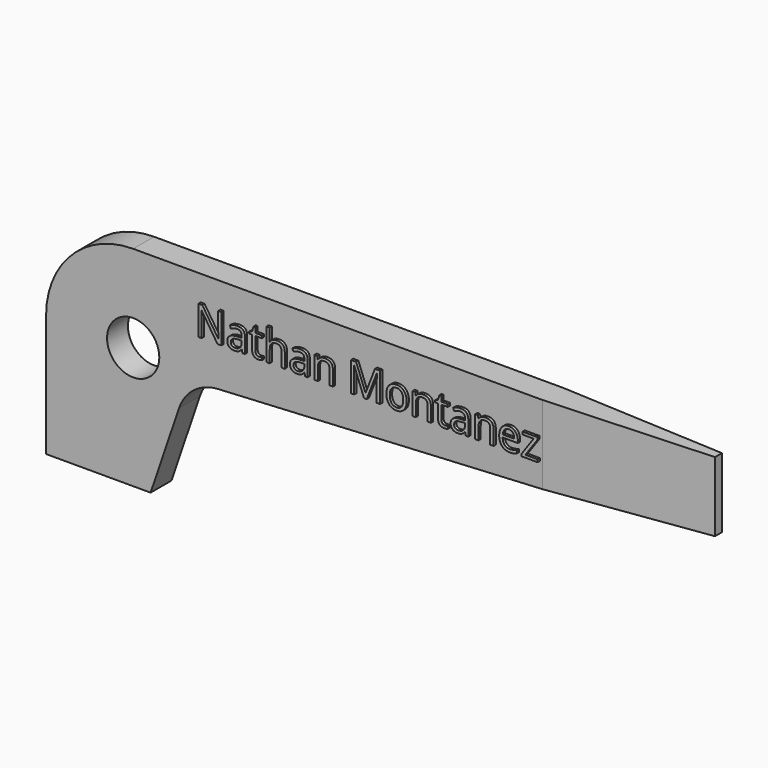
from build123d import *

# Parameters (mm, degrees)
F1_DEPTH     = 2.38125
F2_R         = 2.38125
F3_DEPTH     = 25.4
F5_DEPTH     = 25.4
F6_TEXT_SIZE = 3.7509316959
F7_DEPTH     = 0.254


# Not quite as in the source:
# - Text() gives the source's letters only with a copy of the font that has no kerning and outlines rounded to 1/6400 em; it was checked with that copy


with BuildPart() as f1:
    # F0 (on Front) → F1 (new body)
    with BuildSketch(Plane.XZ):
        with BuildLine():
            Line((60.325, 19.05), (7.9375, 19.05))
            ThreePointArc((7.9375, 19.05), (2.3248399243, 16.7251600757), (0, 11.1125))
            Line((0, 11.1125), (0, 0))
            Line((0, 0), (9.525, 0))
            Line((9.525, 0), (12.1173647876, 7.6271664624))
            ThreePointArc((12.1173647876, 7.6271664624), (13.4786145605, 9.5135918491), (15.6631963617, 10.3130942181))
            Line((15.6631963617, 10.3130942181), (60.325, 12.7))
            Line((60.325, 12.7), (60.325, 19.05))
        make_face()
    extrude(amount=F1_DEPTH)

    # F2 (on face) → F3 (cut)
    with BuildSketch(Plane.XZ.offset(2.38125)):
        with Locations((7.9375, 11.1125)):
            Circle(F2_R)
    extrude(amount=-F3_DEPTH, mode=Mode.SUBTRACT)

    # F4 (on face) → F5 (cut)
    with BuildSketch(Plane.XY.offset(19.05)):
        Polygon((60.325, -2.38125), (60.325, -1.5875), (45.24375, -2.38125), align=None)
        Polygon((60.325, 0), (45.24375, 0), (60.325, -0.79375), align=None)
    extrude(amount=-F5_DEPTH, mode=Mode.SUBTRACT)

    # F6 (on face) → F7 (join)
    with BuildSketch(Plane.XZ.offset(2.38125)):
        with Locations((13.7206855943, 14.079323771)):
            Text('Nathan Montanez', F6_TEXT_SIZE, font='Open Sans', text_align=(TextAlign.LEFT, TextAlign.BOTTOM))
    extrude(amount=F7_DEPTH)


solid = f1.part
